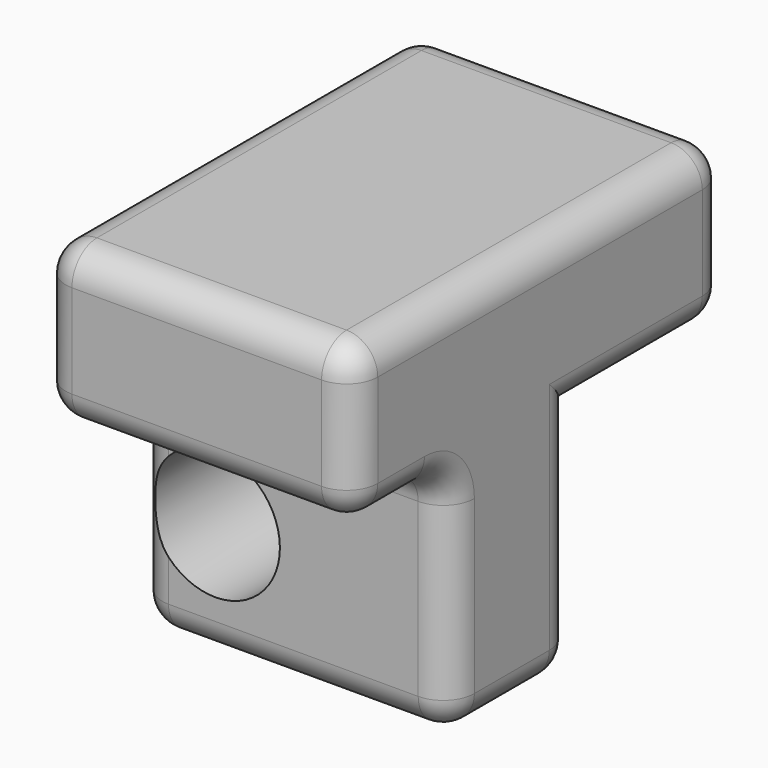
from build123d import *

# Parameters (mm, degrees)
F0_W          = 25.4
F0_H          = 25.4
F1_DEPTH      = 76.2
F2_W          = 25.4
F2_H          = 25.4
F3_DEPTH      = 38.1
F4_R          = 10.5052255275
F5_DEPTH      = 56.5413178334
F7_DEPTH      = 25.4
F8_T1_DEPTH   = 50.8
F8_T3_DEPTH   = 33.02
F8_T5_DEPTH   = 33.02
F8_T7_DEPTH   = 26.0603178334
F8_T9_DEPTH   = 15.24
F8_T11_DEPTH  = 66.04
F8_T13_DEPTH  = 33.02
F8_T15_DEPTH  = 76.2
F8_T17_DEPTH  = 40.64
F8_S21_W      = 5.08
F8_S21_H      = 5.08
F8_T22_DEPTH  = 5.08
F8_S27_W      = 5.08
F8_S27_H      = 5.08
F8_T28_DEPTH  = 5.08
F8_S33_W      = 5.08
F8_S33_H      = 5.08
F8_T34_DEPTH  = 5.08
F8_S39_W      = 5.08
F8_S39_H      = 5.08
F8_T40_DEPTH  = 5.08
F8_S45_W      = 5.08
F8_S45_H      = 5.08
F8_T46_DEPTH  = 5.08
F8_S51_W      = 5.08
F8_S51_H      = 5.08
F8_T52_DEPTH  = 5.08
F8_S57_W      = 5.08
F8_S57_H      = 5.08
F8_T58_DEPTH  = 5.08
F8_S63_W      = 5.08
F8_S63_H      = 5.08
F8_T64_DEPTH  = 5.08
F8_T73_DEPTH  = 45.72
F8_T77_DEPTH  = 38.7603178334
F8_T84_DEPTH  = 45.72
F8_T88_DEPTH  = 38.7603178334
F8_T91_DEPTH  = 27.94
F8_T93_DEPTH  = 9.4996821666
F8_S97_W      = 5.08
F8_S97_H      = 5.08
F8_T98_DEPTH  = 5.08
F8_S103_W     = 5.08
F8_S103_H     = 5.08
F8_T104_DEPTH = 5.08
F8_S109_W     = 5.08
F8_S109_H     = 5.08
F8_T110_DEPTH = 5.08
F8_S115_W     = 5.08
F8_S115_H     = 5.08
F8_T116_DEPTH = 5.08
F8_T120_ANGLE = 90
F8_T122_ANGLE = 90


# Not quite as in the source:
# - a fillet or chamfer that OpenCascade refuses, or shapes differently, is made with other operations: its cross-section is extruded or revolved along the edge and cut away or added


with BuildPart() as f1:
    # F0 (on Front) → F1 (new body)
    with BuildSketch(Plane.XZ):
        with Locations((12.7, 34.7925674498)):
            Rectangle(F0_W, F0_H)
    extrude(amount=F1_DEPTH)

    # F2 (on face) → F3 (join)
    with BuildSketch(Plane(origin=(0, 0, 22.0925674498), x_dir=(1, 0, 0), z_dir=(0, 0, -1))):
        with Locations((12.7, 43.8403178334)):
            Rectangle(F2_W, F2_H)
    extrude(amount=F3_DEPTH)

    # F4 (on face) → F5 (cut, through all)
    with BuildSketch(Plane.XZ.offset(56.5403178334)):
        with Locations((12.7, 3.0425674498)):
            Circle(F4_R)
    extrude(amount=-F5_DEPTH, mode=Mode.SUBTRACT)

    # F6 (on face) → F7 (join)
    with BuildSketch(Plane.YZ.offset(25.4)):
        Polygon((-31.1403178334, -16.0074325502), (-31.1403178334, 22.0925674498), (0, 22.0925674498), (0, 47.4925674498), (-76.2, 47.4925674498), (-76.2, 22.0925674498), (-56.5403178334, 22.0925674498), (-56.5403178334, -16.0074325502), align=None)
    extrude(amount=F7_DEPTH)

    # F8: fillet of radius 5.08 on 24 edges, made by hand

    # F8_s2 → F8_t1 (join)
    with BuildSketch(Plane.YZ):
        with BuildLine():
            ThreePointArc((-61.6203178334, 22.0925674498), (-58.028215385, 20.6046698982), (-56.5403178334, 17.0125674498))
            Line((-56.5403178334, 17.0125674498), (-56.5403178334, 22.0925674498))
            Line((-56.5403178334, 22.0925674498), (-61.6203178334, 22.0925674498))
        make_face()
    extrude(amount=F8_T1_DEPTH)

    # F8_s4 → F8_t3 (cut)
    with BuildSketch(Plane.XZ.offset(36.2203178334)):
        with BuildLine():
            ThreePointArc((50.8, -10.9274325502), (49.3121024484, -14.5195349986), (45.72, -16.0074325502))
            Line((45.72, -16.0074325502), (50.8, -16.0074325502))
            Line((50.8, -16.0074325502), (50.8, -10.9274325502))
        make_face()
        with BuildLine():
            ThreePointArc((0, -10.9274325502), (1.4878975516, -14.5195349986), (5.08, -16.0074325502))
            Line((5.08, -16.0074325502), (0, -16.0074325502))
            Line((0, -16.0074325502), (0, -10.9274325502))
        make_face()
    extrude(amount=F8_T3_DEPTH, mode=Mode.SUBTRACT)

    # F8_s6 → F8_t5 (cut)
    with BuildSketch(Plane.XY.offset(-10.9274325502)):
        with BuildLine():
            ThreePointArc((50.8, -36.2203178334), (49.3121024484, -32.628215385), (45.72, -31.1403178334))
            Line((45.72, -31.1403178334), (50.8, -31.1403178334))
            Line((50.8, -31.1403178334), (50.8, -36.2203178334))
        make_face()
        with BuildLine():
            ThreePointArc((0, -36.2203178334), (1.4878975516, -32.628215385), (5.08, -31.1403178334))
            Line((5.08, -31.1403178334), (0, -31.1403178334))
            Line((0, -31.1403178334), (0, -36.2203178334))
        make_face()
    extrude(amount=F8_T5_DEPTH, mode=Mode.SUBTRACT)

    # F8_s8 → F8_t7 (cut)
    with BuildSketch(Plane.XZ.offset(5.08)):
        with BuildLine():
            ThreePointArc((50.8, 27.1725674498), (49.3121024484, 23.5804650014), (45.72, 22.0925674498))
            Line((45.72, 22.0925674498), (50.8, 22.0925674498))
            Line((50.8, 22.0925674498), (50.8, 27.1725674498))
        make_face()
        with BuildLine():
            ThreePointArc((0, 27.1725674498), (1.4878975516, 23.5804650014), (5.08, 22.0925674498))
            Line((5.08, 22.0925674498), (0, 22.0925674498))
            Line((0, 22.0925674498), (0, 27.1725674498))
        make_face()
    extrude(amount=F8_T7_DEPTH, mode=Mode.SUBTRACT)

    # F8_s10 → F8_t9 (cut)
    with BuildSketch(Plane.XY.offset(27.1725674498)):
        with BuildLine():
            ThreePointArc((45.72, 0), (49.3121024484, -1.4878975516), (50.8, -5.08))
            Line((50.8, -5.08), (50.8, 0))
            Line((50.8, 0), (45.72, 0))
        make_face()
        with BuildLine():
            ThreePointArc((0, -5.08), (1.4878975516, -1.4878975516), (5.08, 0))
            Line((5.08, 0), (0, 0))
            Line((0, 0), (0, -5.08))
        make_face()
    extrude(amount=F8_T9_DEPTH, mode=Mode.SUBTRACT)

    # F8_s12 → F8_t11 (cut)
    with BuildSketch(Plane.XZ.offset(5.08)):
        with BuildLine():
            ThreePointArc((45.72, 47.4925674498), (49.3121024484, 46.0046698982), (50.8, 42.4125674498))
            Line((50.8, 42.4125674498), (50.8, 47.4925674498))
            Line((50.8, 47.4925674498), (45.72, 47.4925674498))
        make_face()
        with BuildLine():
            ThreePointArc((5.08, 47.4925674498), (1.4878975516, 46.0046698982), (0, 42.4125674498))
            Line((0, 42.4125674498), (0, 47.4925674498))
            Line((0, 47.4925674498), (5.08, 47.4925674498))
        make_face()
    extrude(amount=F8_T11_DEPTH, mode=Mode.SUBTRACT)

    # F8_s14 → F8_t13 (cut)
    with BuildSketch(Plane.XY.offset(9.3925674498)):
        with BuildLine():
            ThreePointArc((50.8, -71.12), (49.3121024484, -74.7121024484), (45.72, -76.2))
            Line((45.72, -76.2), (50.8, -76.2))
            Line((50.8, -76.2), (50.8, -71.12))
        make_face()
        with BuildLine():
            ThreePointArc((0, -71.12), (1.4878975516, -74.7121024484), (5.08, -76.2))
            Line((5.08, -76.2), (0, -76.2))
            Line((0, -76.2), (0, -71.12))
        make_face()
    extrude(amount=F8_T13_DEPTH, mode=Mode.SUBTRACT)

    # F8_s16 → F8_t15 (cut)
    with BuildSketch(Plane.YZ.offset(-12.7)):
        with BuildLine():
            ThreePointArc((-56.5403178334, -10.9274325502), (-55.0524202819, -14.5195349986), (-51.4603178334, -16.0074325502))
            Line((-51.4603178334, -16.0074325502), (-56.5403178334, -16.0074325502))
            Line((-56.5403178334, -16.0074325502), (-56.5403178334, -10.9274325502))
        make_face()
        with BuildLine():
            ThreePointArc((-76.2, 27.1725674498), (-74.7121024484, 23.5804650014), (-71.12, 22.0925674498))
            Line((-71.12, 22.0925674498), (-76.2, 22.0925674498))
            Line((-76.2, 22.0925674498), (-76.2, 27.1725674498))
        make_face()
    extrude(amount=F8_T15_DEPTH, mode=Mode.SUBTRACT)

    # F8_s18 → F8_t17 (cut)
    with BuildSketch(Plane.YZ.offset(5.08)):
        with BuildLine():
            ThreePointArc((0, 27.1725674498), (-1.4878975516, 23.5804650014), (-5.08, 22.0925674498))
            Line((-5.08, 22.0925674498), (0, 22.0925674498))
            Line((0, 22.0925674498), (0, 27.1725674498))
        make_face()
        with BuildLine():
            ThreePointArc((-36.2203178334, -16.0074325502), (-32.628215385, -14.5195349986), (-31.1403178334, -10.9274325502))
            Line((-31.1403178334, -10.9274325502), (-31.1403178334, -16.0074325502))
            Line((-31.1403178334, -16.0074325502), (-36.2203178334, -16.0074325502))
        make_face()
        with BuildLine():
            ThreePointArc((-5.08, 47.4925674498), (-1.4878975516, 46.0046698982), (0, 42.4125674498))
            Line((0, 42.4125674498), (0, 47.4925674498))
            Line((0, 47.4925674498), (-5.08, 47.4925674498))
        make_face()
        with BuildLine():
            ThreePointArc((-71.12, 47.4925674498), (-74.7121024484, 46.0046698982), (-76.2, 42.4125674498))
            Line((-76.2, 42.4125674498), (-76.2, 47.4925674498))
            Line((-76.2, 47.4925674498), (-71.12, 47.4925674498))
        make_face()
    extrude(amount=F8_T17_DEPTH, mode=Mode.SUBTRACT)


with BuildPart() as f8_tool20:
    # F8_s21 → F8_t22 (new body)
    with BuildSketch(Plane.XZ.offset(36.2203178334)):
        with Locations((48.26, -13.4674325502)):
            Rectangle(F8_S21_W, F8_S21_H)
    extrude(amount=-F8_T22_DEPTH)

    # F8_s23 → F8_t24 (revolve, cut)
    with BuildSketch(Plane(origin=(45.72, -36.2203178334, -10.9274325502), x_dir=(-0.7071067812, 0, 0.7071067812), z_dir=(-0.7071067812, 0, -0.7071067812))):
        with BuildLine():
            ThreePointArc((0, -5.08), (5.08, 0), (0, 5.08))
            Line((0, 5.08), (0, -5.08))
        make_face()
    revolve(axis=Axis((45.72, -36.2203178334, -10.9274325502), (0, 1, 0)), mode=Mode.SUBTRACT)


with BuildPart() as f1_1:
    add(f1.part)

    # F8_t19: cut F8_tool20
    add(f8_tool20.part, mode=Mode.SUBTRACT)


with BuildPart() as f8_tool26:
    # F8_s27 → F8_t28 (new body)
    with BuildSketch(Plane.XY.offset(27.1725674498)):
        with Locations((48.26, -2.54)):
            Rectangle(F8_S27_W, F8_S27_H)
    extrude(amount=-F8_T28_DEPTH)

    # F8_s29 → F8_t30 (revolve, cut)
    with BuildSketch(Plane(origin=(45.72, -5.08, 27.1725674498), x_dir=(-0.7071067812, -0.7071067812, 0), z_dir=(0.7071067812, -0.7071067812, 0))):
        with BuildLine():
            ThreePointArc((0, -5.08), (5.08, 0), (0, 5.08))
            Line((0, 5.08), (0, -5.08))
        make_face()
    revolve(axis=Axis((45.72, -5.08, 27.1725674498), (0, 0, -1)), mode=Mode.SUBTRACT)


with BuildPart() as f1_2:
    add(f1_1.part)

    # F8_t25: cut F8_tool26
    add(f8_tool26.part, mode=Mode.SUBTRACT)


with BuildPart() as f8_tool32:
    # F8_s33 → F8_t34 (new body)
    with BuildSketch(Plane.XY.offset(42.4125674498)):
        with Locations((48.26, -2.54)):
            Rectangle(F8_S33_W, F8_S33_H)
    extrude(amount=F8_T34_DEPTH)

    # F8_s35 → F8_t36 (revolve, cut)
    with BuildSketch(Plane(origin=(45.72, -5.08, 42.4125674498), x_dir=(-0.7071067812, -0.7071067812, 0), z_dir=(-0.7071067812, 0.7071067812, 0))):
        with BuildLine():
            ThreePointArc((0, -5.08), (5.08, 0), (0, 5.08))
            Line((0, 5.08), (0, -5.08))
        make_face()
    revolve(axis=Axis((45.72, -5.08, 42.4125674498), (0, 0, 1)), mode=Mode.SUBTRACT)


with BuildPart() as f1_3:
    add(f1_2.part)

    # F8_t31: cut F8_tool32
    add(f8_tool32.part, mode=Mode.SUBTRACT)


with BuildPart() as f8_tool38:
    # F8_s39 → F8_t40 (new body)
    with BuildSketch(Plane.XY.offset(42.4125674498)):
        with Locations((48.26, -73.66)):
            Rectangle(F8_S39_W, F8_S39_H)
    extrude(amount=F8_T40_DEPTH)

    # F8_s41 → F8_t42 (revolve, cut)
    with BuildSketch(Plane(origin=(45.72, -71.12, 42.4125674498), x_dir=(-0.7071067812, 0.7071067812, 0), z_dir=(0.7071067812, 0.7071067812, 0))):
        with BuildLine():
            ThreePointArc((0, -5.08), (5.08, 0), (0, 5.08))
            Line((0, 5.08), (0, -5.08))
        make_face()
    revolve(axis=Axis((45.72, -71.12, 42.4125674498), (0, 0, 1)), mode=Mode.SUBTRACT)


with BuildPart() as f1_4:
    add(f1_3.part)

    # F8_t37: cut F8_tool38
    add(f8_tool38.part, mode=Mode.SUBTRACT)


with BuildPart() as f8_tool44:
    # F8_s45 → F8_t46 (new body)
    with BuildSketch(Plane.XY.offset(27.1725674498)):
        with Locations((2.54, -2.54)):
            Rectangle(F8_S45_W, F8_S45_H)
    extrude(amount=-F8_T46_DEPTH)

    # F8_s47 → F8_t48 (revolve, cut)
    with BuildSketch(Plane(origin=(5.08, -5.08, 27.1725674498), x_dir=(0.7071067812, -0.7071067812, 0), z_dir=(0.7071067812, 0.7071067812, 0))):
        with BuildLine():
            ThreePointArc((0, -5.08), (5.08, 0), (0, 5.08))
            Line((0, 5.08), (0, -5.08))
        make_face()
    revolve(axis=Axis((5.08, -5.08, 27.1725674498), (0, 0, -1)), mode=Mode.SUBTRACT)


with BuildPart() as f1_5:
    add(f1_4.part)

    # F8_t43: cut F8_tool44
    add(f8_tool44.part, mode=Mode.SUBTRACT)


with BuildPart() as f8_tool50:
    # F8_s51 → F8_t52 (new body)
    with BuildSketch(Plane.XZ.offset(36.2203178334)):
        with Locations((2.54, -13.4674325502)):
            Rectangle(F8_S51_W, F8_S51_H)
    extrude(amount=-F8_T52_DEPTH)

    # F8_s53 → F8_t54 (revolve, cut)
    with BuildSketch(Plane(origin=(5.08, -36.2203178334, -10.9274325502), x_dir=(0.7071067812, 0, 0.7071067812), z_dir=(-0.7071067812, 0, 0.7071067812))):
        with BuildLine():
            ThreePointArc((0, -5.08), (5.08, 0), (0, 5.08))
            Line((0, 5.08), (0, -5.08))
        make_face()
    revolve(axis=Axis((5.08, -36.2203178334, -10.9274325502), (0, 1, 0)), mode=Mode.SUBTRACT)


with BuildPart() as f1_6:
    add(f1_5.part)

    # F8_t49: cut F8_tool50
    add(f8_tool50.part, mode=Mode.SUBTRACT)


with BuildPart() as f8_tool56:
    # F8_s57 → F8_t58 (new body)
    with BuildSketch(Plane.XY.offset(42.4125674498)):
        with Locations((2.54, -2.54)):
            Rectangle(F8_S57_W, F8_S57_H)
    extrude(amount=F8_T58_DEPTH)

    # F8_s59 → F8_t60 (revolve, cut)
    with BuildSketch(Plane(origin=(5.08, -5.08, 42.4125674498), x_dir=(0.7071067812, -0.7071067812, 0), z_dir=(-0.7071067812, -0.7071067812, 0))):
        with BuildLine():
            ThreePointArc((0, -5.08), (5.08, 0), (0, 5.08))
            Line((0, 5.08), (0, -5.08))
        make_face()
    revolve(axis=Axis((5.08, -5.08, 42.4125674498), (0, 0, 1)), mode=Mode.SUBTRACT)


with BuildPart() as f1_7:
    add(f1_6.part)

    # F8_t55: cut F8_tool56
    add(f8_tool56.part, mode=Mode.SUBTRACT)


with BuildPart() as f8_tool62:
    # F8_s63 → F8_t64 (new body)
    with BuildSketch(Plane.XY.offset(42.4125674498)):
        with Locations((2.54, -73.66)):
            Rectangle(F8_S63_W, F8_S63_H)
    extrude(amount=F8_T64_DEPTH)

    # F8_s65 → F8_t66 (revolve, cut)
    with BuildSketch(Plane(origin=(5.08, -71.12, 42.4125674498), x_dir=(0.7071067812, 0.7071067812, 0), z_dir=(0.7071067812, -0.7071067812, 0))):
        with BuildLine():
            ThreePointArc((0, -5.08), (5.08, 0), (0, 5.08))
            Line((0, 5.08), (0, -5.08))
        make_face()
    revolve(axis=Axis((5.08, -71.12, 42.4125674498), (0, 0, 1)), mode=Mode.SUBTRACT)


with BuildPart() as f1_8:
    add(f1_7.part)

    # F8_t61: cut F8_tool62
    add(f8_tool62.part, mode=Mode.SUBTRACT)

    # F8_s67 → F8_t68 (revolve, cut)
    with BuildSketch(Plane.XY.offset(3.0425674498)):
        with BuildLine():
            ThreePointArc((28.2852255275, -31.1403178334), (24.693123079, -32.628215385), (23.2052255275, -36.2203178334))
            Line((23.2052255275, -36.2203178334), (23.2052255275, -31.1403178334))
            Line((23.2052255275, -31.1403178334), (28.2852255275, -31.1403178334))
        make_face()
    revolve(axis=Axis((12.7, -31.1403178334, 3.0425674498), (0, -1, 0)), mode=Mode.SUBTRACT)


with BuildPart() as f8_tool71:
    # F8_s72 → F8_t73 (new body)
    with BuildSketch(Plane.XY.offset(-10.9274325502)):
        with BuildLine():
            ThreePointArc((50.8, -36.2203178334), (49.3121024484, -32.628215385), (45.72, -31.1403178334))
            Line((45.72, -31.1403178334), (50.8, -31.1403178334))
            Line((50.8, -31.1403178334), (50.8, -36.2203178334))
        make_face()
    extrude(amount=F8_T73_DEPTH)

    split(bisect_by=Plane.XY.offset(22.0925674498), keep=Keep.TOP)


with BuildPart() as f8_tool75:
    # F8_s76 → F8_t77 (new body)
    with BuildSketch(Plane.XZ.offset(43.8403178334)):
        with BuildLine():
            ThreePointArc((50.8, 27.1725674498), (49.3121024484, 23.5804650014), (45.72, 22.0925674498))
            Line((45.72, 22.0925674498), (50.8, 22.0925674498))
            Line((50.8, 22.0925674498), (50.8, 27.1725674498))
        make_face()
    extrude(amount=-F8_T77_DEPTH)

    split(bisect_by=Plane.XZ.offset(31.1403178334), keep=Keep.TOP)


with BuildPart() as f8_tool71_1:
    add(f8_tool71.part)

    # F8_t79: intersect F8_tool75
    add(f8_tool75.part, mode=Mode.INTERSECT)


with BuildPart() as f1_9:
    add(f1_8.part)

    # F8_t69: cut F8_tool71
    add(f8_tool71_1.part, mode=Mode.SUBTRACT)


with BuildPart() as f8_tool82:
    # F8_s83 → F8_t84 (new body)
    with BuildSketch(Plane.XY.offset(34.7925674498)):
        with BuildLine():
            ThreePointArc((0, -36.2203178334), (1.4878975516, -32.628215385), (5.08, -31.1403178334))
            Line((5.08, -31.1403178334), (0, -31.1403178334))
            Line((0, -31.1403178334), (0, -36.2203178334))
        make_face()
    extrude(amount=-F8_T84_DEPTH)

    split(bisect_by=Plane.XY.offset(22.0925674498), keep=Keep.TOP)


with BuildPart() as f8_tool86:
    # F8_s87 → F8_t88 (new body)
    with BuildSketch(Plane.XZ.offset(5.08)):
        with BuildLine():
            ThreePointArc((0, 27.1725674498), (1.4878975516, 23.5804650014), (5.08, 22.0925674498))
            Line((5.08, 22.0925674498), (0, 22.0925674498))
            Line((0, 22.0925674498), (0, 27.1725674498))
        make_face()
    extrude(amount=F8_T88_DEPTH)

    split(bisect_by=Plane.XZ.offset(31.1403178334), keep=Keep.TOP)


with BuildPart() as f8_tool82_1:
    add(f8_tool82.part)

    # F8_t90: intersect F8_tool86
    add(f8_tool86.part, mode=Mode.INTERSECT)


with BuildPart() as f1_10:
    add(f1_9.part)

    # F8_t80: cut F8_tool82
    add(f8_tool82_1.part, mode=Mode.SUBTRACT)

    # F8_s92 → F8_t91 (cut)
    with BuildSketch(Plane.XY.offset(-10.9274325502)):
        with BuildLine():
            ThreePointArc((45.72, -56.5403178334), (49.3121024484, -55.0524202819), (50.8, -51.4603178334))
            Line((50.8, -51.4603178334), (50.8, -56.5403178334))
            Line((50.8, -56.5403178334), (45.72, -56.5403178334))
        make_face()
        with BuildLine():
            ThreePointArc((5.08, -56.5403178334), (1.4878975516, -55.0524202819), (0, -51.4603178334))
            Line((0, -51.4603178334), (0, -56.5403178334))
            Line((0, -56.5403178334), (5.08, -56.5403178334))
        make_face()
    extrude(amount=F8_T91_DEPTH, mode=Mode.SUBTRACT)

    # F8_s94 → F8_t93 (cut)
    with BuildSketch(Plane.XZ.offset(61.6203178334)):
        with BuildLine():
            ThreePointArc((45.72, 22.0925674498), (49.3121024484, 23.5804650014), (50.8, 27.1725674498))
            Line((50.8, 27.1725674498), (50.8, 22.0925674498))
            Line((50.8, 22.0925674498), (45.72, 22.0925674498))
        make_face()
        with BuildLine():
            ThreePointArc((5.08, 22.0925674498), (1.4878975516, 23.5804650014), (0, 27.1725674498))
            Line((0, 27.1725674498), (0, 22.0925674498))
            Line((0, 22.0925674498), (5.08, 22.0925674498))
        make_face()
    extrude(amount=F8_T93_DEPTH, mode=Mode.SUBTRACT)


with BuildPart() as f8_tool96:
    # F8_s97 → F8_t98 (new body)
    with BuildSketch(Plane.XZ.offset(51.4603178334)):
        with Locations((2.54, -13.4674325502)):
            Rectangle(F8_S97_W, F8_S97_H)
    extrude(amount=F8_T98_DEPTH)

    # F8_s99 → F8_t100 (revolve, cut)
    with BuildSketch(Plane(origin=(5.08, -51.4603178334, -10.9274325502), x_dir=(0.7071067812, 0, 0.7071067812), z_dir=(0.7071067812, 0, -0.7071067812))):
        with BuildLine():
            ThreePointArc((0, -5.08), (5.08, 0), (0, 5.08))
            Line((0, 5.08), (0, -5.08))
        make_face()
    revolve(axis=Axis((5.08, -51.4603178334, -10.9274325502), (0, -1, 0)), mode=Mode.SUBTRACT)


with BuildPart() as f1_11:
    add(f1_10.part)

    # F8_t95: cut F8_tool96
    add(f8_tool96.part, mode=Mode.SUBTRACT)


with BuildPart() as f8_tool102:
    # F8_s103 → F8_t104 (new body)
    with BuildSketch(Plane.XY.offset(27.1725674498)):
        with Locations((2.54, -73.66)):
            Rectangle(F8_S103_W, F8_S103_H)
    extrude(amount=-F8_T104_DEPTH)

    # F8_s105 → F8_t106 (revolve, cut)
    with BuildSketch(Plane(origin=(5.08, -71.12, 27.1725674498), x_dir=(0.7071067812, 0.7071067812, 0), z_dir=(-0.7071067812, 0.7071067812, 0))):
        with BuildLine():
            ThreePointArc((0, -5.08), (5.08, 0), (0, 5.08))
            Line((0, 5.08), (0, -5.08))
        make_face()
    revolve(axis=Axis((5.08, -71.12, 27.1725674498), (0, 0, -1)), mode=Mode.SUBTRACT)


with BuildPart() as f1_12:
    add(f1_11.part)

    # F8_t101: cut F8_tool102
    add(f8_tool102.part, mode=Mode.SUBTRACT)


with BuildPart() as f8_tool108:
    # F8_s109 → F8_t110 (new body)
    with BuildSketch(Plane.XY.offset(27.1725674498)):
        with Locations((48.26, -73.66)):
            Rectangle(F8_S109_W, F8_S109_H)
    extrude(amount=-F8_T110_DEPTH)

    # F8_s111 → F8_t112 (revolve, cut)
    with BuildSketch(Plane(origin=(45.72, -71.12, 27.1725674498), x_dir=(-0.7071067812, 0.7071067812, 0), z_dir=(-0.7071067812, -0.7071067812, 0))):
        with BuildLine():
            ThreePointArc((0, -5.08), (5.08, 0), (0, 5.08))
            Line((0, 5.08), (0, -5.08))
        make_face()
    revolve(axis=Axis((45.72, -71.12, 27.1725674498), (0, 0, -1)), mode=Mode.SUBTRACT)


with BuildPart() as f1_13:
    add(f1_12.part)

    # F8_t107: cut F8_tool108
    add(f8_tool108.part, mode=Mode.SUBTRACT)


with BuildPart() as f8_tool114:
    # F8_s115 → F8_t116 (new body)
    with BuildSketch(Plane.XZ.offset(51.4603178334)):
        with Locations((48.26, -13.4674325502)):
            Rectangle(F8_S115_W, F8_S115_H)
    extrude(amount=F8_T116_DEPTH)

    # F8_s117 → F8_t118 (revolve, cut)
    with BuildSketch(Plane(origin=(45.72, -51.4603178334, -10.9274325502), x_dir=(-0.7071067812, 0, 0.7071067812), z_dir=(0.7071067812, 0, 0.7071067812))):
        with BuildLine():
            ThreePointArc((0, -5.08), (5.08, 0), (0, 5.08))
            Line((0, 5.08), (0, -5.08))
        make_face()
    revolve(axis=Axis((45.72, -51.4603178334, -10.9274325502), (0, -1, 0)), mode=Mode.SUBTRACT)


with BuildPart() as f1_14:
    add(f1_13.part)

    # F8_t113: cut F8_tool114
    add(f8_tool114.part, mode=Mode.SUBTRACT)

    # F8_s119 → F8_t120 (revolve, cut)
    with BuildSketch(Plane.XZ.offset(61.6203178334)):
        with BuildLine():
            ThreePointArc((5.08, 22.0925674498), (1.4878975516, 23.5804650014), (0, 27.1725674498))
            Line((0, 27.1725674498), (0, 22.0925674498))
            Line((0, 22.0925674498), (5.08, 22.0925674498))
        make_face()
    revolve(axis=Axis((0, -61.6203178334, 17.0125674498), (-1, 0, 0)), revolution_arc=F8_T120_ANGLE, mode=Mode.SUBTRACT)

    # F8_s121 → F8_t122 (revolve, cut)
    with BuildSketch(Plane.XZ.offset(61.6203178334)):
        with BuildLine():
            ThreePointArc((45.72, 22.0925674498), (49.3121024484, 23.5804650014), (50.8, 27.1725674498))
            Line((50.8, 27.1725674498), (50.8, 22.0925674498))
            Line((50.8, 22.0925674498), (45.72, 22.0925674498))
        make_face()
    revolve(axis=Axis((50.8, -61.6203178334, 17.0125674498), (-1, 0, 0)), revolution_arc=F8_T122_ANGLE, mode=Mode.SUBTRACT)


solid = f1_14.part
